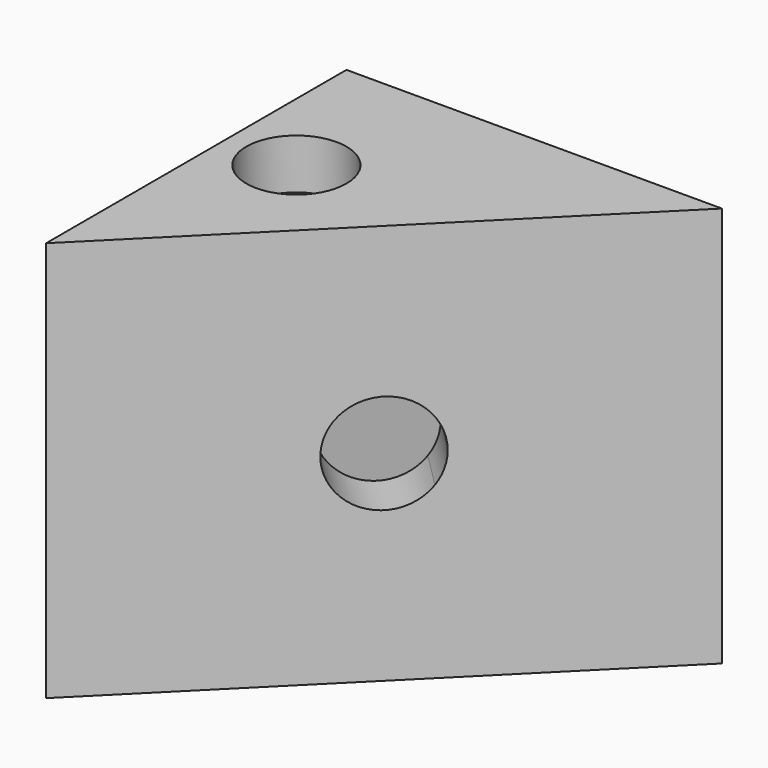
from build123d import *

# Parameters (mm, degrees)
F1_DEPTH = 25.4
F2_T     = -3.175
F3_DEPTH = 25.4
F5_DEPTH = 3.175
F6_R     = 3.175
F7_DEPTH = 25.4
F9_DEPTH = 3.175


# Not quite as in the source:
# - a feature names something its author has since deleted; it is built from what else it names


with BuildPart() as f1:
    # F0 (on Top) → F1 (new body)
    with BuildSketch(Plane.XY):
        Polygon((11.90625, 11.90625), (-11.90625, 11.90625), (-11.90625, -11.90625), align=None)
    extrude(amount=F1_DEPTH)

    # F2
    f2_openings = [f1.faces().sort_by_distance(p)[0] for p in [
        (-11.90625, 0, 12.7),
    ]]
    offset(amount=F2_T, openings=f2_openings)

    # F3 (cut): a face of the model
    f3_faces = [f1.faces().sort_by_distance(p)[0] for p in [
        (-6.5237926868, 3.3487926868, 3.175),
    ]]
    extrude(f3_faces, amount=-F3_DEPTH, mode=Mode.SUBTRACT)

    # F4 (on face) → F5 (cut)
    with BuildSketch(Plane(origin=(-11.90625, 0, 0), x_dir=(0, -1, 0), z_dir=(-1, 0, 0))):
        with BuildLine():
            ThreePointArc((3.175, 12.7), (2.9133467904, 13.962155093), (2.1715130842, 15.0162806231))
            Line((2.1715130842, 15.0162806231), (0, 12.7))
            Line((0, 12.7), (2.1715130842, 10.3837193769))
            ThreePointArc((2.1715130842, 10.3837193769), (2.9133467904, 11.437844907), (3.175, 12.7))
        make_face()
        with BuildLine():
            Line((0, 12.7), (2.1715130842, 15.0162806231))
            ThreePointArc((2.1715130842, 15.0162806231), (0, 15.875), (-2.1715130842, 15.0162806231))
            Line((-2.1715130842, 15.0162806231), (0, 12.7))
        make_face()
        with BuildLine():
            Line((-2.1715130842, 10.3837193769), (0, 12.7))
            Line((0, 12.7), (-2.1715130842, 15.0162806231))
            ThreePointArc((-2.1715130842, 15.0162806231), (-3.175, 12.7), (-2.1715130842, 10.3837193769))
        make_face()
        with BuildLine():
            Line((2.1715130842, 10.3837193769), (0, 12.7))
            Line((0, 12.7), (-2.1715130842, 10.3837193769))
            ThreePointArc((-2.1715130842, 10.3837193769), (0, 9.525), (2.1715130842, 10.3837193769))
        make_face()
    extrude(amount=-F5_DEPTH, mode=Mode.SUBTRACT)

    # F6 (on face) → F7 (cut)
    with BuildSketch(Plane.XY.offset(25.4)):
        with Locations((-7.46125, 2.38125)):
            Circle(F6_R)
    extrude(amount=-F7_DEPTH, mode=Mode.SUBTRACT)

    # F8 (on face) → F9 (cut)
    with BuildSketch(Plane(origin=(0, 0, 0), x_dir=(0.7071067812, 0.7071067812, 0), z_dir=(0.7071067812, -0.7071067812, 0))):
        with BuildLine():
            ThreePointArc((3.175, 12.7), (1.0081076412, 15.7107048982), (-2.5348229819, 14.6118832209))
            Line((-2.5348229819, 14.6118832209), (2.5348229819, 10.7881167791))
            ThreePointArc((2.5348229819, 10.7881167791), (3.0107048982, 11.6918923588), (3.175, 12.7))
        make_face()
        with BuildLine():
            Line((2.5348229819, 10.7881167791), (-2.5348229819, 14.6118832209))
            ThreePointArc((-2.5348229819, 14.6118832209), (-1.9118832209, 10.1651770181), (2.5348229819, 10.7881167791))
        make_face()
    extrude(amount=-F9_DEPTH, mode=Mode.SUBTRACT)


solid = f1.part
